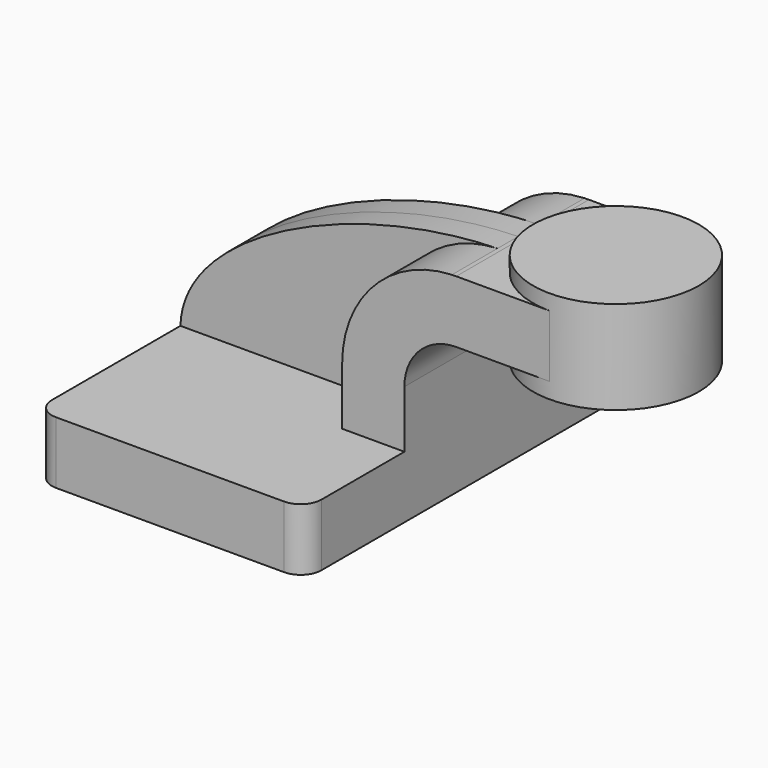
from build123d import *

# Parameters (mm, degrees)
F1_DEPTH = 63.5
F2_DEPTH = 25.4
F3_DEPTH = 7.9375
F5_R     = 6.35


# Not quite as in the source:
# - a feature names something its author has since deleted; it is built from what else it names


with BuildPart() as f1:
    # F0 (on Front) → F1 (new body, symmetric)
    with BuildSketch(Plane.XZ):
        Polygon((22.225, 9.525), (-41.275, 9.525), (-41.275, -9.525), (41.275, -9.525), (41.275, 9.525), align=None)
    extrude(amount=F1_DEPTH, both=True)

    # F0 (on Front) → F2 (join, symmetric)
    with BuildSketch(Plane.XZ):
        with BuildLine():
            Line((85.725, 61.9848461288), (60.325, 61.9848461288))
            Line((60.325, 61.9848461288), (57.15, 61.9848461288))
            add(Edge.make_bspline(
                [(55.8188394438, 61.9594684272), (56.2631889725, 61.9701778386), (56.7069273587, 61.9786434716), (57.15, 61.9848461288)],
                knots=[110.4431341751, 110.4431341751, 110.4431341751, 110.4431341751, 111.5325785628, 111.5325785628, 111.5325785628, 111.5325785628], degree=3))
            ThreePointArc((55.8188394438, 61.9594684272), (31.9880604143, 51.2803420215), (22.225, 27.0598461288))
            Line((22.225, 27.0598461288), (22.225, 9.525))
            Line((22.225, 9.525), (41.275, 9.525))
            Line((41.275, 9.525), (41.275, 27.0598461288))
            ThreePointArc((41.275, 27.0598461288), (45.9246798487, 38.2851662801), (57.15, 42.9348461288))
            Line((57.15, 42.9348461288), (60.325, 42.9348461288))
            Line((60.325, 42.9348461288), (85.725, 42.9348461288))
            Line((85.725, 42.9348461288), (85.725, 61.9848461288))
        make_face()
    extrude(amount=F2_DEPTH, both=True)

    # F0 (on Front) → F3 (join, symmetric)
    with BuildSketch(Plane.XZ):
        with BuildLine():
            ThreePointArc((22.225, 27.0598461288), (31.9880604143, 51.2803420215), (55.8188394438, 61.9594684272))
            add(Edge.make_bspline(
                [(-41.275, 9.525), (-40.5543307974, 36.728759834), (10.7726166473, 60.8737948733), (55.8188394438, 61.9594684272)],
                knots=[0, 0, 0, 0, 110.4431341751, 110.4431341751, 110.4431341751, 110.4431341751], degree=3))
            Line((-41.275, 9.525), (22.225, 9.525))
            Line((22.225, 9.525), (22.225, 27.0598461288))
        make_face()
    extrude(amount=F3_DEPTH, both=True)

    # F0 (on Front) → F4 (revolve)
    with BuildSketch(Plane.XZ):
        Polygon((111.125, 66.675), (85.725, 66.675), (85.725, 61.9848461288), (85.725, 42.9348461288), (85.725, 38.1), (111.125, 38.1), align=None)
    revolve(axis=Axis((85.725, 0, 52.3875), (0, 0, 1)))

    # F5
    f5_edges = [f1.edges().sort_by_distance(p)[0] for p in [
        (41.275, -63.5, 0),
        (-41.275, -63.5, 0),
        (-41.275, 63.5, 0),
        (41.275, 63.5, 0),
    ]]
    fillet(f5_edges, radius=F5_R)


solid = f1.part
